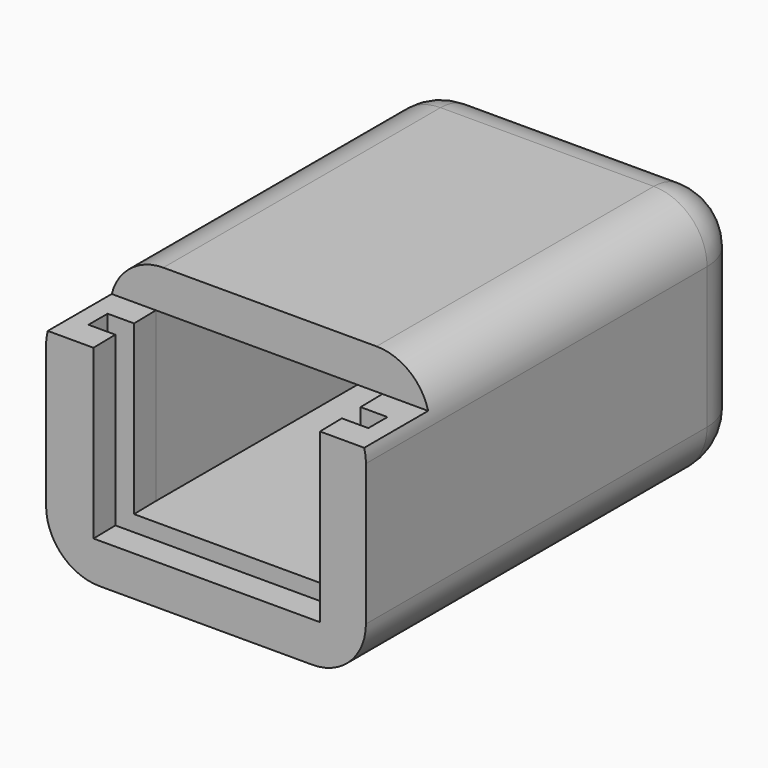
from build123d import *

# Parameters (mm, degrees)
F0_W         = 8.5
F0_H         = 13.5
F0_W_2       = 1.7211329822
F0_H_2       = 1.5
F0_W_3       = 1.7788670178
F1_DEPTH     = 0.9
F2_DEPTH     = 1.5
F3_DEPTH     = 7.8
F5_W         = 12
F5_H         = 15
F6_DEPTH     = 1.5
F7_R         = 3
F8_DEPTH     = 16.501
F9_T1_DEPTH  = 5.3
F9_T3_DEPTH  = 8
F9_T5_DEPTH  = 18
F9_T7_DEPTH  = 21
F9_S11_W     = 2
F9_S11_H     = 2
F9_T12_DEPTH = 2
F9_S17_W     = 2
F9_S17_H     = 2
F9_T18_DEPTH = 2
F9_S23_W     = 2
F9_S23_H     = 2
F9_T24_DEPTH = 2
F9_S29_W     = 2
F9_S29_H     = 2
F9_T30_DEPTH = 2


# Not quite as in the source:
# - a fillet or chamfer that OpenCascade refuses, or shapes differently, is made with other operations: its cross-section is extruded or revolved along the edge and cut away or added
# - a feature names something its author has since deleted; it is built from what else it names


with BuildPart() as f1:
    # F0 (on Top) → F1 (new body)
    with BuildSketch(Plane.XY):
        with Locations((-0.0288670178, 8.25)):
            Rectangle(F0_W, F0_H)
        Polygon((-6, 1.5), (-6, -1.5), (-4.2211329822, -1.5), (-4.2413398946, -0.45), (-5.25, -0.45), (-5.25, 0.45), (-4.2586601054, 0.45), (-4.2788670178, 1.5), align=None)
        Polygon((4.2211329822, 1.5), (-4.2788670178, 1.5), (-4.2586601054, 0.45), (4.2413398946, 0.45), align=None)
        with Locations((-5.1394335089, 8.25)):
            Rectangle(F0_W_2, F0_H)
        Polygon((4.2586601054, -0.45), (4.2788670178, -1.5), (6, -1.5), (6, 1.5), (4.2211329822, 1.5), (4.2413398946, 0.45), (5.25, 0.45), (5.25, -0.45), align=None)
        Polygon((-4.2413398946, -0.45), (-4.2211329822, -1.5), (4.2788670178, -1.5), (4.2586601054, -0.45), align=None)
        Polygon((-4.2586601054, 0.45), (-4.2413398946, -0.45), (4.2586601054, -0.45), (4.2413398946, 0.45), align=None)
        Polygon((-5.25, -0.45), (-4.2413398946, -0.45), (-4.2586601054, 0.45), (-5.25, 0.45), align=None)
        Polygon((4.2413398946, 0.45), (4.2586601054, -0.45), (5.25, -0.45), (5.25, 0.45), align=None)
        with Locations((-5.1394335089, 15.75)):
            Rectangle(F0_W_2, F0_H_2)
        with Locations((-0.0288670178, 15.75)):
            Rectangle(F0_W, F0_H_2)
        with Locations((5.1105664911, 15.75)):
            Rectangle(F0_W_3, F0_H_2)
        with Locations((5.1105664911, 8.25)):
            Rectangle(F0_W_3, F0_H)
    extrude(amount=F1_DEPTH)

    # F0 (on Top) → F2 (join)
    with BuildSketch(Plane.XY):
        Polygon((-4.2413398946, -0.45), (-4.2211329822, -1.5), (4.2788670178, -1.5), (4.2586601054, -0.45), align=None)
        Polygon((-6, 1.5), (-6, -1.5), (-4.2211329822, -1.5), (-4.2413398946, -0.45), (-5.25, -0.45), (-5.25, 0.45), (-4.2586601054, 0.45), (-4.2788670178, 1.5), align=None)
        Polygon((4.2586601054, -0.45), (4.2788670178, -1.5), (6, -1.5), (6, 1.5), (4.2211329822, 1.5), (4.2413398946, 0.45), (5.25, 0.45), (5.25, -0.45), align=None)
        Polygon((4.2211329822, 1.5), (-4.2788670178, 1.5), (-4.2586601054, 0.45), (4.2413398946, 0.45), align=None)
        with Locations((-5.1394335089, 8.25)):
            Rectangle(F0_W_2, F0_H)
        with Locations((5.1105664911, 8.25)):
            Rectangle(F0_W_3, F0_H)
        with Locations((-0.0288670178, 8.25)):
            Rectangle(F0_W, F0_H)
        with Locations((-5.1394335089, 15.75)):
            Rectangle(F0_W_2, F0_H_2)
        with Locations((-0.0288670178, 15.75)):
            Rectangle(F0_W, F0_H_2)
        with Locations((5.1105664911, 15.75)):
            Rectangle(F0_W_3, F0_H_2)
    extrude(amount=F2_DEPTH)

    # F0 (on Top) → F3 (join)
    with BuildSketch(Plane.XY):
        Polygon((-6, 1.5), (-6, -1.5), (-4.2211329822, -1.5), (-4.2413398946, -0.45), (-5.25, -0.45), (-5.25, 0.45), (-4.2586601054, 0.45), (-4.2788670178, 1.5), align=None)
        Polygon((4.2586601054, -0.45), (4.2788670178, -1.5), (6, -1.5), (6, 1.5), (4.2211329822, 1.5), (4.2413398946, 0.45), (5.25, 0.45), (5.25, -0.45), align=None)
        with Locations((-5.1394335089, 8.25)):
            Rectangle(F0_W_2, F0_H)
        with Locations((5.1105664911, 8.25)):
            Rectangle(F0_W_3, F0_H)
        with Locations((-5.1394335089, 15.75)):
            Rectangle(F0_W_2, F0_H_2)
        with Locations((-0.0288670178, 15.75)):
            Rectangle(F0_W, F0_H_2)
        with Locations((5.1105664911, 15.75)):
            Rectangle(F0_W_3, F0_H_2)
    extrude(amount=F3_DEPTH)

    # F5 (on offset) → F6 (join)
    with BuildSketch(Plane.XY.offset(7.8)):
        with Locations((0, 9)):
            Rectangle(F5_W, F5_H)
    extrude(amount=F6_DEPTH)

    # F7 (on Front) → F8 (cut, through all)
    with BuildSketch(Plane.XZ):
        with Locations((0, 4.5)):
            Circle(F7_R)
    extrude(amount=-F8_DEPTH, mode=Mode.SUBTRACT)

    # F9: fillet of radius 2 on 8 edges, made by hand

    # F9_s2 → F9_t1 (cut)
    with BuildSketch(Plane.XY.offset(2)):
        with BuildLine():
            ThreePointArc((4, 16.5), (5.4142135624, 15.9142135624), (6, 14.5))
            Line((6, 14.5), (6, 16.5))
            Line((6, 16.5), (4, 16.5))
        make_face()
        with BuildLine():
            ThreePointArc((-4, 16.5), (-5.4142135624, 15.9142135624), (-6, 14.5))
            Line((-6, 14.5), (-6, 16.5))
            Line((-6, 16.5), (-4, 16.5))
        make_face()
    extrude(amount=F9_T1_DEPTH, mode=Mode.SUBTRACT)

    # F9_s4 → F9_t3 (cut)
    with BuildSketch(Plane.YZ.offset(-4)):
        with BuildLine():
            ThreePointArc((16.5, 7.3), (15.9142135624, 8.7142135624), (14.5, 9.3))
            Line((14.5, 9.3), (16.5, 9.3))
            Line((16.5, 9.3), (16.5, 7.3))
        make_face()
        with BuildLine():
            ThreePointArc((14.5, 0), (15.9142135624, 0.5857864376), (16.5, 2))
            Line((16.5, 2), (16.5, 0))
            Line((16.5, 0), (14.5, 0))
        make_face()
    extrude(amount=F9_T3_DEPTH, mode=Mode.SUBTRACT)

    # F9_s6 → F9_t5 (cut)
    with BuildSketch(Plane.XZ.offset(-14.5)):
        with BuildLine():
            ThreePointArc((4, 9.3), (5.4142135624, 8.7142135624), (6, 7.3))
            Line((6, 7.3), (6, 9.3))
            Line((6, 9.3), (4, 9.3))
        make_face()
        with BuildLine():
            ThreePointArc((-4, 9.3), (-5.4142135624, 8.7142135624), (-6, 7.3))
            Line((-6, 7.3), (-6, 9.3))
            Line((-6, 9.3), (-4, 9.3))
        make_face()
    extrude(amount=F9_T5_DEPTH, mode=Mode.SUBTRACT)

    # F9_s8 → F9_t7 (cut)
    with BuildSketch(Plane.XZ.offset(-14.5)):
        with BuildLine():
            ThreePointArc((4, 0), (5.4142135624, 0.5857864376), (6, 2))
            Line((6, 2), (6, 0))
            Line((6, 0), (4, 0))
        make_face()
        with BuildLine():
            ThreePointArc((-4, 0), (-5.4142135624, 0.5857864376), (-6, 2))
            Line((-6, 2), (-6, 0))
            Line((-6, 0), (-4, 0))
        make_face()
    extrude(amount=F9_T7_DEPTH, mode=Mode.SUBTRACT)


with BuildPart() as f9_tool10:
    # F9_s11 → F9_t12 (new body)
    with BuildSketch(Plane.XY.offset(2)):
        with Locations((5, 15.5)):
            Rectangle(F9_S11_W, F9_S11_H)
    extrude(amount=-F9_T12_DEPTH)

    # F9_s13 → F9_t14 (revolve, cut)
    with BuildSketch(Plane(origin=(4, 14.5, 2), x_dir=(-0.7071067812, -0.7071067812, 0), z_dir=(0.7071067812, -0.7071067812, 0))):
        with BuildLine():
            ThreePointArc((0, -2), (2, 0), (0, 2))
            Line((0, 2), (0, -2))
        make_face()
    revolve(axis=Axis((4, 14.5, 2), (0, 0, -1)), mode=Mode.SUBTRACT)


with BuildPart() as f1_1:
    add(f1.part)

    # F9_t9: cut F9_tool10
    add(f9_tool10.part, mode=Mode.SUBTRACT)


with BuildPart() as f9_tool16:
    # F9_s17 → F9_t18 (new body)
    with BuildSketch(Plane.XY.offset(7.3)):
        with Locations((5, 15.5)):
            Rectangle(F9_S17_W, F9_S17_H)
    extrude(amount=F9_T18_DEPTH)

    # F9_s19 → F9_t20 (revolve, cut)
    with BuildSketch(Plane(origin=(4, 14.5, 7.3), x_dir=(-0.7071067812, -0.7071067812, 0), z_dir=(-0.7071067812, 0.7071067812, 0))):
        with BuildLine():
            ThreePointArc((0, -2), (2, 0), (0, 2))
            Line((0, 2), (0, -2))
        make_face()
    revolve(axis=Axis((4, 14.5, 7.3), (0, 0, 1)), mode=Mode.SUBTRACT)


with BuildPart() as f1_2:
    add(f1_1.part)

    # F9_t15: cut F9_tool16
    add(f9_tool16.part, mode=Mode.SUBTRACT)


with BuildPart() as f9_tool22:
    # F9_s23 → F9_t24 (new body)
    with BuildSketch(Plane.YZ.offset(-4)):
        with Locations((15.5, 8.3)):
            Rectangle(F9_S23_W, F9_S23_H)
    extrude(amount=-F9_T24_DEPTH)

    # F9_s25 → F9_t26 (revolve, cut)
    with BuildSketch(Plane(origin=(-4, 14.5, 7.3), x_dir=(0, -0.7071067812, -0.7071067812), z_dir=(0, 0.7071067812, -0.7071067812))):
        with BuildLine():
            ThreePointArc((0, -2), (2, 0), (0, 2))
            Line((0, 2), (0, -2))
        make_face()
    revolve(axis=Axis((-4, 14.5, 7.3), (-1, 0, 0)), mode=Mode.SUBTRACT)


with BuildPart() as f1_3:
    add(f1_2.part)

    # F9_t21: cut F9_tool22
    add(f9_tool22.part, mode=Mode.SUBTRACT)


with BuildPart() as f9_tool28:
    # F9_s29 → F9_t30 (new body)
    with BuildSketch(Plane.YZ.offset(-4)):
        with Locations((15.5, 1)):
            Rectangle(F9_S29_W, F9_S29_H)
    extrude(amount=-F9_T30_DEPTH)

    # F9_s31 → F9_t32 (revolve, cut)
    with BuildSketch(Plane(origin=(-4, 14.5, 2), x_dir=(0, -0.7071067812, 0.7071067812), z_dir=(0, -0.7071067812, -0.7071067812))):
        with BuildLine():
            ThreePointArc((0, -2), (2, 0), (0, 2))
            Line((0, 2), (0, -2))
        make_face()
    revolve(axis=Axis((-4, 14.5, 2), (-1, 0, 0)), mode=Mode.SUBTRACT)


with BuildPart() as f1_4:
    add(f1_3.part)

    # F9_t27: cut F9_tool28
    add(f9_tool28.part, mode=Mode.SUBTRACT)


solid = f1_4.part
